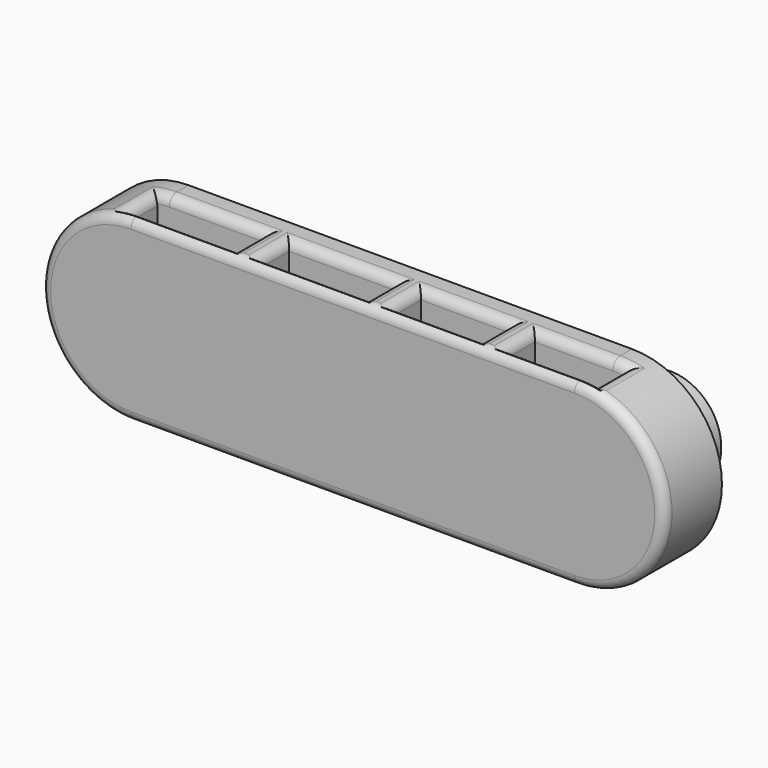
from build123d import *

# Parameters (mm, degrees)
F0_R          = 2.9
F1_DEPTH      = 2
F2_DEPTH      = 6
F3_W          = 9
F3_H          = 3
F3_W_2        = 7.5
F3_W_3        = 1
F3_W_4        = 8
F3_W_5        = 6.5
F4_DEPTH      = 15.001
F5_R          = 4.25
F5_R_2        = 2.9
F6_DEPTH      = 2
F7_T1_DEPTH   = 3
F7_T3_DEPTH   = 6.5
F7_T5_DEPTH   = 7.5
F7_T7_DEPTH   = 9
F7_T9_DEPTH   = 8
F7_T11_DEPTH  = 37
F7_T14_ANGLE  = 180
F7_T18_ANGLE  = 22.9411746719
F7_T21_ANGLE  = 180
F7_T25_ANGLE  = 22.9411746719
F7_T30_ANGLE  = 22.9411746719
F7_T35_ANGLE  = 22.9411746719
F7_T40_ANGLE  = 22.9411746719
F7_T45_ANGLE  = 22.9411746719
F7_T50_ANGLE  = 22.9411746719
F7_T55_ANGLE  = 22.9411746719
F7_T61_DEPTH  = 5.5904344641
F7_T66_ANGLE  = 22.9411746719
F7_T73_ANGLE  = 22.9411746719
F7_T77_DEPTH  = 5.5904344641
F7_T85_ANGLE  = 22.9411746719
F7_T89_DEPTH  = 5.5904344641
F7_T97_DEPTH  = 5.5904344641
F7_T102_ANGLE = 22.9411746719
F7_T109_DEPTH = 5
F7_T113_DEPTH = 8.5
F7_T120_DEPTH = 8.5
F7_T124_DEPTH = 5
F7_T132_DEPTH = 5
F7_T137_DEPTH = 9.5
F7_T144_DEPTH = 5
F7_T148_DEPTH = 9.5
F7_T155_DEPTH = 5
F7_T159_DEPTH = 9.5
F7_T166_DEPTH = 9.5
F7_T170_DEPTH = 5
F7_T178_DEPTH = 5
F7_T183_DEPTH = 11
F7_T190_DEPTH = 5
F7_T194_DEPTH = 11
F7_T201_DEPTH = 5
F7_T205_DEPTH = 11
F7_T212_DEPTH = 11
F7_T216_DEPTH = 5
F7_T224_DEPTH = 5
F7_T229_DEPTH = 10
F7_T236_DEPTH = 10
F7_T240_DEPTH = 5
F7_T247_DEPTH = 5.5904344641
F7_T252_ANGLE = 22.9411746719
F7_T259_ANGLE = 22.9411746719
F7_T263_DEPTH = 5.5904344641
F7_T271_ANGLE = 22.9411746719
F7_T275_DEPTH = 5.5904344641
F7_T283_DEPTH = 5.5904344641
F7_T288_ANGLE = 22.9411746719
F7_T295_DEPTH = 5
F7_T300_DEPTH = 8.5
F7_T307_DEPTH = 8.5
F7_T311_DEPTH = 5
F7_T318_DEPTH = 9.5
F7_T322_DEPTH = 5
F7_T330_DEPTH = 9.5
F7_T334_DEPTH = 5
F7_T341_DEPTH = 9.5
F7_T345_DEPTH = 5
F7_T352_DEPTH = 5
F7_T357_DEPTH = 9.5
F7_T364_DEPTH = 11
F7_T368_DEPTH = 5
F7_T376_DEPTH = 11
F7_T380_DEPTH = 5
F7_T387_DEPTH = 11
F7_T391_DEPTH = 5
F7_T398_DEPTH = 5
F7_T403_DEPTH = 11
F7_T410_DEPTH = 10
F7_T414_DEPTH = 5
F7_T422_DEPTH = 5
F7_T426_DEPTH = 10


# Not quite as in the source:
# - a fillet or chamfer that OpenCascade refuses, or shapes differently, is made with other operations: its cross-section is extruded or revolved along the edge and cut away or added


with BuildPart() as f1:
    # F0 (on Front) → F1 (new body)
    with BuildSketch(Plane.XZ):
        with Locations((-18.5, 0)):
            Circle(F0_R)
    extrude(amount=-F1_DEPTH)



with BuildPart() as f1b:
    # F0 (on Front) → F1, piece 2 (new body)
    with BuildSketch(Plane.XZ):
        with Locations((18.5, 0)):
            Circle(F0_R)
    extrude(amount=-F1_DEPTH)


with BuildPart() as f1_1:
    add(f1.part)

    add(f1b.part)  # F2 merges F1b
    # F0 (on Front) → F2 (join)
    with BuildSketch(Plane.XZ):
        with BuildLine():
            Line((18.5, 7.5), (-18.5, 7.5))
            ThreePointArc((-18.5, 7.5), (-26, 0), (-18.5, -7.5))
            Line((-18.5, -7.5), (18.5, -7.5))
            ThreePointArc((18.5, -7.5), (26, 0), (18.5, 7.5))
        make_face()
        with Locations((-18.5, 0)):
            Circle(F0_R, mode=Mode.SUBTRACT)
        with Locations((18.5, 0)):
            Circle(F0_R, mode=Mode.SUBTRACT)
        with Locations((-18.5, 0)):
            Circle(F0_R)
        with Locations((18.5, 0)):
            Circle(F0_R)
    extrude(amount=F2_DEPTH)

    # F3 (on face) → F4 (cut, through all)
    with BuildSketch(Plane.XY.offset(7.5)):
        with Locations((-4, -3.5)):
            Rectangle(F3_W, F3_H)
        with Locations((6.25, -3.5)):
            Rectangle(F3_W_2, F3_H)
        with Locations((-19, -3.5)):
            Rectangle(F3_W_3, F3_H)
        with Locations((-14.5, -3.5)):
            Rectangle(F3_W_4, F3_H)
        with Locations((15.25, -3.5)):
            Rectangle(F3_W_5, F3_H)
        with Locations((19, -3.5)):
            Rectangle(F3_W_3, F3_H)
    extrude(amount=-F4_DEPTH, mode=Mode.SUBTRACT)

    # F5 (on face) → F6 (join)
    with BuildSketch(Plane(origin=(0, 2, 0), x_dir=(-1, 0, 0), z_dir=(0, 1, 0))):
        with Locations((-18.5, 0)):
            Circle(F5_R)
        with Locations((18.5, 0)):
            Circle(F5_R)
        with Locations((18.5, 0)):
            Circle(F5_R_2, mode=Mode.SUBTRACT)
        with Locations((18.5, 0)):
            Circle(F5_R_2)
    extrude(amount=F6_DEPTH)

    # F7: fillet of radius 0.8 on 40 edges, made by hand

    # F7_s2 → F7_t1 (cut)
    with BuildSketch(Plane.XZ.offset(2)):
        with BuildLine():
            ThreePointArc((20.5149253731, 7.2242699106), (19.8162336817, 7.0908389885), (19.5, 6.4536811201))
            Line((19.5, 6.4536811201), (19.5, 7.4330343737))
            ThreePointArc((19.5, 7.4330343737), (20.0110722688, 7.3462004192), (20.5149253731, 7.2242699106))
        make_face()
        with BuildLine():
            ThreePointArc((20.5149253731, -7.2242699106), (19.8162336817, -7.0908389885), (19.5, -6.4536811201))
            Line((19.5, -6.4536811201), (19.5, -7.4330343737))
            ThreePointArc((19.5, -7.4330343737), (20.0110722688, -7.3462004192), (20.5149253731, -7.2242699106))
        make_face()
        with BuildLine():
            ThreePointArc((11.2, 7.5), (11.7656854249, 7.2656854249), (12, 6.7))
            Line((12, 6.7), (12, 7.5))
            Line((12, 7.5), (11.2, 7.5))
        make_face()
        with BuildLine():
            ThreePointArc((10.8, 7.5), (10.2343145751, 7.2656854249), (10, 6.7))
            Line((10, 6.7), (10, 7.5))
            Line((10, 7.5), (10.8, 7.5))
        make_face()
        with BuildLine():
            ThreePointArc((1.7, 7.5), (2.2656854249, 7.2656854249), (2.5, 6.7))
            Line((2.5, 6.7), (2.5, 7.5))
            Line((2.5, 7.5), (1.7, 7.5))
        make_face()
        with BuildLine():
            ThreePointArc((1.3, 7.5), (0.7343145751, 7.2656854249), (0.5, 6.7))
            Line((0.5, 6.7), (0.5, 7.5))
            Line((0.5, 7.5), (1.3, 7.5))
        make_face()
        with BuildLine():
            ThreePointArc((-9.3, 7.5), (-8.7343145751, 7.2656854249), (-8.5, 6.7))
            Line((-8.5, 6.7), (-8.5, 7.5))
            Line((-8.5, 7.5), (-9.3, 7.5))
        make_face()
        with BuildLine():
            ThreePointArc((-9.7, 7.5), (-10.2656854249, 7.2656854249), (-10.5, 6.7))
            Line((-10.5, 6.7), (-10.5, 7.5))
            Line((-10.5, 7.5), (-9.7, 7.5))
        make_face()
        with BuildLine():
            ThreePointArc((-20.5149253731, -7.2242699106), (-19.8162336817, -7.0908389885), (-19.5, -6.4536811201))
            Line((-19.5, -6.4536811201), (-19.5, -7.4330343737))
            ThreePointArc((-19.5, -7.4330343737), (-20.0110722688, -7.3462004192), (-20.5149253731, -7.2242699106))
        make_face()
        with BuildLine():
            ThreePointArc((-20.5149253731, 7.2242699106), (-19.8162336817, 7.0908389885), (-19.5, 6.4536811201))
            Line((-19.5, 6.4536811201), (-19.5, 7.4330343737))
            ThreePointArc((-19.5, 7.4330343737), (-20.0110722688, 7.3462004192), (-20.5149253731, 7.2242699106))
        make_face()
        with BuildLine():
            ThreePointArc((11.2, -7.5), (11.7656854249, -7.2656854249), (12, -6.7))
            Line((12, -6.7), (12, -7.5))
            Line((12, -7.5), (11.2, -7.5))
        make_face()
        with BuildLine():
            ThreePointArc((10.8, -7.5), (10.2343145751, -7.2656854249), (10, -6.7))
            Line((10, -6.7), (10, -7.5))
            Line((10, -7.5), (10.8, -7.5))
        make_face()
        with BuildLine():
            ThreePointArc((1.7, -7.5), (2.2656854249, -7.2656854249), (2.5, -6.7))
            Line((2.5, -6.7), (2.5, -7.5))
            Line((2.5, -7.5), (1.7, -7.5))
        make_face()
        with BuildLine():
            ThreePointArc((1.3, -7.5), (0.7343145751, -7.2656854249), (0.5, -6.7))
            Line((0.5, -6.7), (0.5, -7.5))
            Line((0.5, -7.5), (1.3, -7.5))
        make_face()
        with BuildLine():
            ThreePointArc((-9.3, -7.5), (-8.7343145751, -7.2656854249), (-8.5, -6.7))
            Line((-8.5, -6.7), (-8.5, -7.5))
            Line((-8.5, -7.5), (-9.3, -7.5))
        make_face()
        with BuildLine():
            ThreePointArc((-9.7, -7.5), (-10.2656854249, -7.2656854249), (-10.5, -6.7))
            Line((-10.5, -6.7), (-10.5, -7.5))
            Line((-10.5, -7.5), (-9.7, -7.5))
        make_face()
    extrude(amount=F7_T1_DEPTH, mode=Mode.SUBTRACT)

    # F7_s4 → F7_t3 (cut)
    with BuildSketch(Plane.YZ.offset(12)):
        with BuildLine():
            ThreePointArc((-5.8, 7.5), (-5.2343145751, 7.2656854249), (-5, 6.7))
            Line((-5, 6.7), (-5, 7.5))
            Line((-5, 7.5), (-5.8, 7.5))
        make_face()
        with BuildLine():
            ThreePointArc((-1.2, 7.5), (-1.7656854249, 7.2656854249), (-2, 6.7))
            Line((-2, 6.7), (-2, 7.5))
            Line((-2, 7.5), (-1.2, 7.5))
        make_face()
        with BuildLine():
            ThreePointArc((-5.8, -7.5), (-5.2343145751, -7.2656854249), (-5, -6.7))
            Line((-5, -6.7), (-5, -7.5))
            Line((-5, -7.5), (-5.8, -7.5))
        make_face()
        with BuildLine():
            ThreePointArc((-1.2, -7.5), (-1.7656854249, -7.2656854249), (-2, -6.7))
            Line((-2, -6.7), (-2, -7.5))
            Line((-2, -7.5), (-1.2, -7.5))
        make_face()
    extrude(amount=F7_T3_DEPTH, mode=Mode.SUBTRACT)

    # F7_s6 → F7_t5 (cut)
    with BuildSketch(Plane.YZ.offset(2.5)):
        with BuildLine():
            ThreePointArc((-5.8, 7.5), (-5.2343145751, 7.2656854249), (-5, 6.7))
            Line((-5, 6.7), (-5, 7.5))
            Line((-5, 7.5), (-5.8, 7.5))
        make_face()
        with BuildLine():
            ThreePointArc((-1.2, 7.5), (-1.7656854249, 7.2656854249), (-2, 6.7))
            Line((-2, 6.7), (-2, 7.5))
            Line((-2, 7.5), (-1.2, 7.5))
        make_face()
        with BuildLine():
            ThreePointArc((-1.2, -7.5), (-1.7656854249, -7.2656854249), (-2, -6.7))
            Line((-2, -6.7), (-2, -7.5))
            Line((-2, -7.5), (-1.2, -7.5))
        make_face()
        with BuildLine():
            ThreePointArc((-5.8, -7.5), (-5.2343145751, -7.2656854249), (-5, -6.7))
            Line((-5, -6.7), (-5, -7.5))
            Line((-5, -7.5), (-5.8, -7.5))
        make_face()
    extrude(amount=F7_T5_DEPTH, mode=Mode.SUBTRACT)

    # F7_s8 → F7_t7 (cut)
    with BuildSketch(Plane.YZ.offset(-8.5)):
        with BuildLine():
            ThreePointArc((-1.2, 7.5), (-1.7656854249, 7.2656854249), (-2, 6.7))
            Line((-2, 6.7), (-2, 7.5))
            Line((-2, 7.5), (-1.2, 7.5))
        make_face()
        with BuildLine():
            ThreePointArc((-5.8, 7.5), (-5.2343145751, 7.2656854249), (-5, 6.7))
            Line((-5, 6.7), (-5, 7.5))
            Line((-5, 7.5), (-5.8, 7.5))
        make_face()
        with BuildLine():
            ThreePointArc((-1.2, -7.5), (-1.7656854249, -7.2656854249), (-2, -6.7))
            Line((-2, -6.7), (-2, -7.5))
            Line((-2, -7.5), (-1.2, -7.5))
        make_face()
        with BuildLine():
            ThreePointArc((-5.8, -7.5), (-5.2343145751, -7.2656854249), (-5, -6.7))
            Line((-5, -6.7), (-5, -7.5))
            Line((-5, -7.5), (-5.8, -7.5))
        make_face()
    extrude(amount=F7_T7_DEPTH, mode=Mode.SUBTRACT)

    # F7_s10 → F7_t9 (cut)
    with BuildSketch(Plane.YZ.offset(-18.5)):
        with BuildLine():
            ThreePointArc((-5.8, 7.5), (-5.2343145751, 7.2656854249), (-5, 6.7))
            Line((-5, 6.7), (-5, 7.5))
            Line((-5, 7.5), (-5.8, 7.5))
        make_face()
        with BuildLine():
            ThreePointArc((-1.2, 7.5), (-1.7656854249, 7.2656854249), (-2, 6.7))
            Line((-2, 6.7), (-2, 7.5))
            Line((-2, 7.5), (-1.2, 7.5))
        make_face()
        with BuildLine():
            ThreePointArc((-1.2, -7.5), (-1.7656854249, -7.2656854249), (-2, -6.7))
            Line((-2, -6.7), (-2, -7.5))
            Line((-2, -7.5), (-1.2, -7.5))
        make_face()
        with BuildLine():
            ThreePointArc((-5.8, -7.5), (-5.2343145751, -7.2656854249), (-5, -6.7))
            Line((-5, -6.7), (-5, -7.5))
            Line((-5, -7.5), (-5.8, -7.5))
        make_face()
    extrude(amount=F7_T9_DEPTH, mode=Mode.SUBTRACT)

    # F7_s12 → F7_t11 (cut)
    with BuildSketch(Plane.YZ.offset(-18.5)):
        with BuildLine():
            ThreePointArc((-5.2, 7.5), (-5.7656854249, 7.2656854249), (-6, 6.7))
            Line((-6, 6.7), (-6, 7.5))
            Line((-6, 7.5), (-5.2, 7.5))
        make_face()
        with BuildLine():
            ThreePointArc((-5.2, -7.5), (-5.7656854249, -7.2656854249), (-6, -6.7))
            Line((-6, -6.7), (-6, -7.5))
            Line((-6, -7.5), (-5.2, -7.5))
        make_face()
    extrude(amount=F7_T11_DEPTH, mode=Mode.SUBTRACT)

    # F7_s13 → F7_t14 (revolve, cut)
    with BuildSketch(Plane.YZ.offset(-18.5)):
        with BuildLine():
            ThreePointArc((-5.2, 7.5), (-5.7656854249, 7.2656854249), (-6, 6.7))
            Line((-6, 6.7), (-6, 7.5))
            Line((-6, 7.5), (-5.2, 7.5))
        make_face()
    revolve(axis=Axis((-18.5, -6, 0), (0, -1, 0)), revolution_arc=F7_T14_ANGLE, mode=Mode.SUBTRACT)


with BuildPart() as f7_tool16:
    # F7_s17 → F7_t18 (revolve)
    with BuildSketch(Plane.YZ.offset(18.5)):
        with BuildLine():
            ThreePointArc((-1.2, 7.5), (-1.7656854249, 7.2656854249), (-2, 6.7))
            Line((-2, 6.7), (-2, 7.5))
            Line((-2, 7.5), (-1.2, 7.5))
        make_face()
    revolve(axis=Axis((18.5, -2, 0), (0, 1, 0)), revolution_arc=F7_T18_ANGLE)

    split(bisect_by=Plane.YZ.offset(19.5), keep=Keep.BOTTOM)


with BuildPart() as f1_2:
    add(f1_1.part)

    # F7_t15: cut F7_tool16
    add(f7_tool16.part, mode=Mode.SUBTRACT)

    # F7_s20 → F7_t21 (revolve, cut)
    with BuildSketch(Plane.YZ.offset(18.5)):
        with BuildLine():
            ThreePointArc((-5.2, -7.5), (-5.7656854249, -7.2656854249), (-6, -6.7))
            Line((-6, -6.7), (-6, -7.5))
            Line((-6, -7.5), (-5.2, -7.5))
        make_face()
    revolve(axis=Axis((18.5, -6, 0), (0, -1, 0)), revolution_arc=F7_T21_ANGLE, mode=Mode.SUBTRACT)


with BuildPart() as f7_tool23:
    # F7_s24 → F7_t25 (revolve)
    with BuildSketch(Plane(origin=(15.6892394171, 0, 6.640684884), x_dir=(0, 1, 0), z_dir=(0.9209055302, 0, 0.3897858444))):
        with BuildLine():
            ThreePointArc((-1.2, -14.7110381211), (-1.7656854249, -14.476723546), (-2, -13.9110381211))
            Line((-2, -13.9110381211), (-2, -14.7110381211))
            Line((-2, -14.7110381211), (-1.2, -14.7110381211))
        make_face()
    revolve(axis=Axis((18.5, -2, 0), (0, 1, 0)), revolution_arc=F7_T25_ANGLE)

    split(bisect_by=Plane.YZ.offset(19.5), keep=Keep.BOTTOM)


with BuildPart() as f1_3:
    add(f1_2.part)

    # F7_t22: cut F7_tool23
    add(f7_tool23.part, mode=Mode.SUBTRACT)


with BuildPart() as f7_tool28:
    # F7_s29 → F7_t30 (revolve)
    with BuildSketch(Plane.YZ.offset(-18.5)):
        with BuildLine():
            ThreePointArc((-1.2, -7.5), (-1.7656854249, -7.2656854249), (-2, -6.7))
            Line((-2, -6.7), (-2, -7.5))
            Line((-2, -7.5), (-1.2, -7.5))
        make_face()
    revolve(axis=Axis((-18.5, -2, 0), (0, 1, 0)), revolution_arc=F7_T30_ANGLE)

    split(bisect_by=Plane.YZ.offset(-19.5), keep=Keep.TOP)


with BuildPart() as f1_4:
    add(f1_3.part)

    # F7_t27: cut F7_tool28
    add(f7_tool28.part, mode=Mode.SUBTRACT)


with BuildPart() as f7_tool33:
    # F7_s34 → F7_t35 (revolve)
    with BuildSketch(Plane(origin=(-15.6892394171, 0, -6.640684884), x_dir=(0, 1, 0), z_dir=(-0.9209055302, 0, -0.3897858444))):
        with BuildLine():
            ThreePointArc((-1.2, -14.7110381211), (-1.7656854249, -14.476723546), (-2, -13.9110381211))
            Line((-2, -13.9110381211), (-2, -14.7110381211))
            Line((-2, -14.7110381211), (-1.2, -14.7110381211))
        make_face()
    revolve(axis=Axis((-18.5, -2, 0), (0, 1, 0)), revolution_arc=F7_T35_ANGLE)

    split(bisect_by=Plane.YZ.offset(-19.5), keep=Keep.TOP)


with BuildPart() as f1_5:
    add(f1_4.part)

    # F7_t32: cut F7_tool33
    add(f7_tool33.part, mode=Mode.SUBTRACT)


with BuildPart() as f7_tool38:
    # F7_s39 → F7_t40 (revolve)
    with BuildSketch(Plane.YZ.offset(-18.5)):
        with BuildLine():
            ThreePointArc((-5.8, -7.5), (-5.2343145751, -7.2656854249), (-5, -6.7))
            Line((-5, -6.7), (-5, -7.5))
            Line((-5, -7.5), (-5.8, -7.5))
        make_face()
    revolve(axis=Axis((-18.5, -5, 0), (0, 1, 0)), revolution_arc=F7_T40_ANGLE)

    split(bisect_by=Plane.YZ.offset(-19.5), keep=Keep.TOP)


with BuildPart() as f1_6:
    add(f1_5.part)

    # F7_t37: cut F7_tool38
    add(f7_tool38.part, mode=Mode.SUBTRACT)


with BuildPart() as f7_tool43:
    # F7_s44 → F7_t45 (revolve)
    with BuildSketch(Plane(origin=(15.6892394171, 0, 6.640684884), x_dir=(0, 1, 0), z_dir=(0.9209055302, 0, 0.3897858444))):
        with BuildLine():
            ThreePointArc((-5.8, -14.7110381211), (-5.2343145751, -14.476723546), (-5, -13.9110381211))
            Line((-5, -13.9110381211), (-5, -14.7110381211))
            Line((-5, -14.7110381211), (-5.8, -14.7110381211))
        make_face()
    revolve(axis=Axis((18.5, -5, 0), (0, 1, 0)), revolution_arc=F7_T45_ANGLE)

    split(bisect_by=Plane.YZ.offset(19.5), keep=Keep.BOTTOM)


with BuildPart() as f1_7:
    add(f1_6.part)

    # F7_t42: cut F7_tool43
    add(f7_tool43.part, mode=Mode.SUBTRACT)


with BuildPart() as f7_tool48:
    # F7_s49 → F7_t50 (revolve)
    with BuildSketch(Plane(origin=(-15.6892394171, 0, -6.640684884), x_dir=(0, 1, 0), z_dir=(-0.9209055302, 0, -0.3897858444))):
        with BuildLine():
            ThreePointArc((-5.8, -14.7110381211), (-5.2343145751, -14.476723546), (-5, -13.9110381211))
            Line((-5, -13.9110381211), (-5, -14.7110381211))
            Line((-5, -14.7110381211), (-5.8, -14.7110381211))
        make_face()
    revolve(axis=Axis((-18.5, -5, 0), (0, 1, 0)), revolution_arc=F7_T50_ANGLE)

    split(bisect_by=Plane.YZ.offset(-19.5), keep=Keep.TOP)


with BuildPart() as f1_8:
    add(f1_7.part)

    # F7_t47: cut F7_tool48
    add(f7_tool48.part, mode=Mode.SUBTRACT)


with BuildPart() as f7_tool53:
    # F7_s54 → F7_t55 (revolve)
    with BuildSketch(Plane.YZ.offset(18.5)):
        with BuildLine():
            ThreePointArc((-5.8, 7.5), (-5.2343145751, 7.2656854249), (-5, 6.7))
            Line((-5, 6.7), (-5, 7.5))
            Line((-5, 7.5), (-5.8, 7.5))
        make_face()
    revolve(axis=Axis((18.5, -5, 0), (0, 1, 0)), revolution_arc=F7_T55_ANGLE)

    split(bisect_by=Plane.YZ.offset(19.5), keep=Keep.BOTTOM)


with BuildPart() as f1_9:
    add(f1_8.part)

    # F7_t52: cut F7_tool53
    add(f7_tool53.part, mode=Mode.SUBTRACT)


with BuildPart() as f7_tool59:
    # F7_s60 → F7_t61 (new body)
    with BuildSketch(Plane.XZ.offset(7.5904344641)):
        with BuildLine():
            ThreePointArc((20.5149253731, 7.2242699106), (19.8162336817, 7.0908389885), (19.5, 6.4536811201))
            Line((19.5, 6.4536811201), (19.5, 7.4330343737))
            ThreePointArc((19.5, 7.4330343737), (20.0110722688, 7.3462004192), (20.5149253731, 7.2242699106))
        make_face()
    extrude(amount=-F7_T61_DEPTH)

    split(bisect_by=Plane.XZ.offset(6), keep=Keep.BOTTOM)

    split(bisect_by=Plane.XZ.offset(5), keep=Keep.TOP)


with BuildPart() as f7_tool64:
    # F7_s65 → F7_t66 (revolve)
    with BuildSketch(Plane.YZ.offset(18.5)):
        with BuildLine():
            ThreePointArc((-5.8, 7.5), (-5.2343145751, 7.2656854249), (-5, 6.7))
            Line((-5, 6.7), (-5, 7.5))
            Line((-5, 7.5), (-5.8, 7.5))
        make_face()
    revolve(axis=Axis((18.5, -5, 0), (0, 1, 0)), revolution_arc=F7_T66_ANGLE)

    split(bisect_by=Plane.YZ.offset(19.5), keep=Keep.TOP)


with BuildPart() as f7_tool59_1:
    add(f7_tool59.part)

    # F7_t68: intersect F7_tool64
    add(f7_tool64.part, mode=Mode.INTERSECT)


with BuildPart() as f1_10:
    add(f1_9.part)

    # F7_t57: cut F7_tool59
    add(f7_tool59_1.part, mode=Mode.SUBTRACT)


with BuildPart() as f7_tool71:
    # F7_s72 → F7_t73 (revolve)
    with BuildSketch(Plane.YZ.offset(18.5)):
        with BuildLine():
            ThreePointArc((-1.2, 7.5), (-1.7656854249, 7.2656854249), (-2, 6.7))
            Line((-2, 6.7), (-2, 7.5))
            Line((-2, 7.5), (-1.2, 7.5))
        make_face()
    revolve(axis=Axis((18.5, -2, 0), (0, 1, 0)), revolution_arc=F7_T73_ANGLE)

    split(bisect_by=Plane.YZ.offset(19.5), keep=Keep.TOP)


with BuildPart() as f7_tool75:
    # F7_s76 → F7_t77 (new body)
    with BuildSketch(Plane.XZ.offset(5)):
        with BuildLine():
            ThreePointArc((20.5149253731, 7.2242699106), (19.8162336817, 7.0908389885), (19.5, 6.4536811201))
            Line((19.5, 6.4536811201), (19.5, 7.4330343737))
            ThreePointArc((19.5, 7.4330343737), (20.0110722688, 7.3462004192), (20.5149253731, 7.2242699106))
        make_face()
    extrude(amount=-F7_T77_DEPTH)

    split(bisect_by=Plane.XZ, keep=Keep.TOP)

    split(bisect_by=Plane.XZ.offset(2), keep=Keep.BOTTOM)


with BuildPart() as f7_tool71_1:
    add(f7_tool71.part)

    # F7_t80: intersect F7_tool75
    add(f7_tool75.part, mode=Mode.INTERSECT)


with BuildPart() as f1_11:
    add(f1_10.part)

    # F7_t69: cut F7_tool71
    add(f7_tool71_1.part, mode=Mode.SUBTRACT)


with BuildPart() as f7_tool83:
    # F7_s84 → F7_t85 (revolve)
    with BuildSketch(Plane(origin=(15.6892394171, 0, 6.640684884), x_dir=(0, 1, 0), z_dir=(0.9209055302, 0, 0.3897858444))):
        with BuildLine():
            ThreePointArc((-5.8, -14.7110381211), (-5.2343145751, -14.476723546), (-5, -13.9110381211))
            Line((-5, -13.9110381211), (-5, -14.7110381211))
            Line((-5, -14.7110381211), (-5.8, -14.7110381211))
        make_face()
    revolve(axis=Axis((18.5, -5, 0), (0, 1, 0)), revolution_arc=F7_T85_ANGLE)

    split(bisect_by=Plane.YZ.offset(19.5), keep=Keep.TOP)


with BuildPart() as f7_tool87:
    # F7_s88 → F7_t89 (new body)
    with BuildSketch(Plane.XZ.offset(7.5904344641)):
        with BuildLine():
            ThreePointArc((20.5149253731, -7.2242699106), (19.8162336817, -7.0908389885), (19.5, -6.4536811201))
            Line((19.5, -6.4536811201), (19.5, -7.4330343737))
            ThreePointArc((19.5, -7.4330343737), (20.0110722688, -7.3462004192), (20.5149253731, -7.2242699106))
        make_face()
    extrude(amount=-F7_T89_DEPTH)

    split(bisect_by=Plane.XZ.offset(6), keep=Keep.BOTTOM)

    split(bisect_by=Plane.XZ.offset(5), keep=Keep.TOP)


with BuildPart() as f7_tool83_1:
    add(f7_tool83.part)

    # F7_t92: intersect F7_tool87
    add(f7_tool87.part, mode=Mode.INTERSECT)


with BuildPart() as f1_12:
    add(f1_11.part)

    # F7_t81: cut F7_tool83
    add(f7_tool83_1.part, mode=Mode.SUBTRACT)


with BuildPart() as f7_tool95:
    # F7_s96 → F7_t97 (new body)
    with BuildSketch(Plane.XZ.offset(5)):
        with BuildLine():
            ThreePointArc((20.5149253731, -7.2242699106), (19.8162336817, -7.0908389885), (19.5, -6.4536811201))
            Line((19.5, -6.4536811201), (19.5, -7.4330343737))
            ThreePointArc((19.5, -7.4330343737), (20.0110722688, -7.3462004192), (20.5149253731, -7.2242699106))
        make_face()
    extrude(amount=-F7_T97_DEPTH)

    split(bisect_by=Plane.XZ, keep=Keep.TOP)

    split(bisect_by=Plane.XZ.offset(2), keep=Keep.BOTTOM)


with BuildPart() as f7_tool100:
    # F7_s101 → F7_t102 (revolve)
    with BuildSketch(Plane(origin=(15.6892394171, 0, 6.640684884), x_dir=(0, 1, 0), z_dir=(0.9209055302, 0, 0.3897858444))):
        with BuildLine():
            ThreePointArc((-1.2, -14.7110381211), (-1.7656854249, -14.476723546), (-2, -13.9110381211))
            Line((-2, -13.9110381211), (-2, -14.7110381211))
            Line((-2, -14.7110381211), (-1.2, -14.7110381211))
        make_face()
    revolve(axis=Axis((18.5, -2, 0), (0, 1, 0)), revolution_arc=F7_T102_ANGLE)

    split(bisect_by=Plane.YZ.offset(19.5), keep=Keep.TOP)


with BuildPart() as f7_tool95_1:
    add(f7_tool95.part)

    # F7_t104: intersect F7_tool100
    add(f7_tool100.part, mode=Mode.INTERSECT)


with BuildPart() as f1_13:
    add(f1_12.part)

    # F7_t93: cut F7_tool95
    add(f7_tool95_1.part, mode=Mode.SUBTRACT)


with BuildPart() as f7_tool107:
    # F7_s108 → F7_t109 (new body)
    with BuildSketch(Plane.XZ):
        with BuildLine():
            ThreePointArc((11.2, 7.5), (11.7656854249, 7.2656854249), (12, 6.7))
            Line((12, 6.7), (12, 7.5))
            Line((12, 7.5), (11.2, 7.5))
        make_face()
    extrude(amount=F7_T109_DEPTH)

    split(bisect_by=Plane.XZ.offset(2), keep=Keep.BOTTOM)


with BuildPart() as f7_tool111:
    # F7_s112 → F7_t113 (new body)
    with BuildSketch(Plane.YZ.offset(18.5)):
        with BuildLine():
            ThreePointArc((-1.2, 7.5), (-1.7656854249, 7.2656854249), (-2, 6.7))
            Line((-2, 6.7), (-2, 7.5))
            Line((-2, 7.5), (-1.2, 7.5))
        make_face()
    extrude(amount=-F7_T113_DEPTH)

    split(bisect_by=Plane.YZ.offset(12), keep=Keep.BOTTOM)


with BuildPart() as f7_tool107_1:
    add(f7_tool107.part)

    # F7_t115: intersect F7_tool111
    add(f7_tool111.part, mode=Mode.INTERSECT)


with BuildPart() as f1_14:
    add(f1_13.part)

    # F7_t105: cut F7_tool107
    add(f7_tool107_1.part, mode=Mode.SUBTRACT)


with BuildPart() as f7_tool118:
    # F7_s119 → F7_t120 (new body)
    with BuildSketch(Plane.YZ.offset(10)):
        with BuildLine():
            ThreePointArc((-5.8, 7.5), (-5.2343145751, 7.2656854249), (-5, 6.7))
            Line((-5, 6.7), (-5, 7.5))
            Line((-5, 7.5), (-5.8, 7.5))
        make_face()
    extrude(amount=F7_T120_DEPTH)

    split(bisect_by=Plane.YZ.offset(12), keep=Keep.BOTTOM)


with BuildPart() as f7_tool122:
    # F7_s123 → F7_t124 (new body)
    with BuildSketch(Plane.XZ.offset(2)):
        with BuildLine():
            ThreePointArc((11.2, 7.5), (11.7656854249, 7.2656854249), (12, 6.7))
            Line((12, 6.7), (12, 7.5))
            Line((12, 7.5), (11.2, 7.5))
        make_face()
    extrude(amount=F7_T124_DEPTH)

    split(bisect_by=Plane.XZ.offset(6), keep=Keep.BOTTOM)

    split(bisect_by=Plane.XZ.offset(5), keep=Keep.TOP)


with BuildPart() as f7_tool118_1:
    add(f7_tool118.part)

    # F7_t127: intersect F7_tool122
    add(f7_tool122.part, mode=Mode.INTERSECT)


with BuildPart() as f1_15:
    add(f1_14.part)

    # F7_t116: cut F7_tool118
    add(f7_tool118_1.part, mode=Mode.SUBTRACT)


with BuildPart() as f7_tool130:
    # F7_s131 → F7_t132 (new body)
    with BuildSketch(Plane.XZ.offset(7)):
        with BuildLine():
            ThreePointArc((10.8, 7.5), (10.2343145751, 7.2656854249), (10, 6.7))
            Line((10, 6.7), (10, 7.5))
            Line((10, 7.5), (10.8, 7.5))
        make_face()
    extrude(amount=-F7_T132_DEPTH)

    split(bisect_by=Plane.XZ.offset(6), keep=Keep.BOTTOM)

    split(bisect_by=Plane.XZ.offset(5), keep=Keep.TOP)


with BuildPart() as f7_tool135:
    # F7_s136 → F7_t137 (new body)
    with BuildSketch(Plane.YZ.offset(2.5)):
        with BuildLine():
            ThreePointArc((-5.8, 7.5), (-5.2343145751, 7.2656854249), (-5, 6.7))
            Line((-5, 6.7), (-5, 7.5))
            Line((-5, 7.5), (-5.8, 7.5))
        make_face()
    extrude(amount=F7_T137_DEPTH)

    split(bisect_by=Plane.YZ.offset(10), keep=Keep.TOP)


with BuildPart() as f7_tool130_1:
    add(f7_tool130.part)

    # F7_t139: intersect F7_tool135
    add(f7_tool135.part, mode=Mode.INTERSECT)


with BuildPart() as f1_16:
    add(f1_15.part)

    # F7_t128: cut F7_tool130
    add(f7_tool130_1.part, mode=Mode.SUBTRACT)


with BuildPart() as f7_tool142:
    # F7_s143 → F7_t144 (new body)
    with BuildSketch(Plane.XZ.offset(5)):
        with BuildLine():
            ThreePointArc((10.8, 7.5), (10.2343145751, 7.2656854249), (10, 6.7))
            Line((10, 6.7), (10, 7.5))
            Line((10, 7.5), (10.8, 7.5))
        make_face()
    extrude(amount=-F7_T144_DEPTH)

    split(bisect_by=Plane.XZ.offset(2), keep=Keep.BOTTOM)


with BuildPart() as f7_tool146:
    # F7_s147 → F7_t148 (new body)
    with BuildSketch(Plane.YZ.offset(12)):
        with BuildLine():
            ThreePointArc((-1.2, 7.5), (-1.7656854249, 7.2656854249), (-2, 6.7))
            Line((-2, 6.7), (-2, 7.5))
            Line((-2, 7.5), (-1.2, 7.5))
        make_face()
    extrude(amount=-F7_T148_DEPTH)

    split(bisect_by=Plane.YZ.offset(10), keep=Keep.TOP)


with BuildPart() as f7_tool142_1:
    add(f7_tool142.part)

    # F7_t150: intersect F7_tool146
    add(f7_tool146.part, mode=Mode.INTERSECT)


with BuildPart() as f1_17:
    add(f1_16.part)

    # F7_t140: cut F7_tool142
    add(f7_tool142_1.part, mode=Mode.SUBTRACT)


with BuildPart() as f7_tool153:
    # F7_s154 → F7_t155 (new body)
    with BuildSketch(Plane.XZ):
        with BuildLine():
            ThreePointArc((1.7, 7.5), (2.2656854249, 7.2656854249), (2.5, 6.7))
            Line((2.5, 6.7), (2.5, 7.5))
            Line((2.5, 7.5), (1.7, 7.5))
        make_face()
    extrude(amount=F7_T155_DEPTH)

    split(bisect_by=Plane.XZ.offset(2), keep=Keep.BOTTOM)


with BuildPart() as f7_tool157:
    # F7_s158 → F7_t159 (new body)
    with BuildSketch(Plane.YZ.offset(10)):
        with BuildLine():
            ThreePointArc((-1.2, 7.5), (-1.7656854249, 7.2656854249), (-2, 6.7))
            Line((-2, 6.7), (-2, 7.5))
            Line((-2, 7.5), (-1.2, 7.5))
        make_face()
    extrude(amount=-F7_T159_DEPTH)

    split(bisect_by=Plane.YZ.offset(2.5), keep=Keep.BOTTOM)


with BuildPart() as f7_tool153_1:
    add(f7_tool153.part)

    # F7_t161: intersect F7_tool157
    add(f7_tool157.part, mode=Mode.INTERSECT)


with BuildPart() as f1_18:
    add(f1_17.part)

    # F7_t151: cut F7_tool153
    add(f7_tool153_1.part, mode=Mode.SUBTRACT)


with BuildPart() as f7_tool164:
    # F7_s165 → F7_t166 (new body)
    with BuildSketch(Plane.YZ.offset(0.5)):
        with BuildLine():
            ThreePointArc((-5.8, 7.5), (-5.2343145751, 7.2656854249), (-5, 6.7))
            Line((-5, 6.7), (-5, 7.5))
            Line((-5, 7.5), (-5.8, 7.5))
        make_face()
    extrude(amount=F7_T166_DEPTH)

    split(bisect_by=Plane.YZ.offset(2.5), keep=Keep.BOTTOM)


with BuildPart() as f7_tool168:
    # F7_s169 → F7_t170 (new body)
    with BuildSketch(Plane.XZ.offset(2)):
        with BuildLine():
            ThreePointArc((1.7, 7.5), (2.2656854249, 7.2656854249), (2.5, 6.7))
            Line((2.5, 6.7), (2.5, 7.5))
            Line((2.5, 7.5), (1.7, 7.5))
        make_face()
    extrude(amount=F7_T170_DEPTH)

    split(bisect_by=Plane.XZ.offset(6), keep=Keep.BOTTOM)

    split(bisect_by=Plane.XZ.offset(5), keep=Keep.TOP)


with BuildPart() as f7_tool164_1:
    add(f7_tool164.part)

    # F7_t173: intersect F7_tool168
    add(f7_tool168.part, mode=Mode.INTERSECT)


with BuildPart() as f1_19:
    add(f1_18.part)

    # F7_t162: cut F7_tool164
    add(f7_tool164_1.part, mode=Mode.SUBTRACT)


with BuildPart() as f7_tool176:
    # F7_s177 → F7_t178 (new body)
    with BuildSketch(Plane.XZ.offset(7)):
        with BuildLine():
            ThreePointArc((1.3, 7.5), (0.7343145751, 7.2656854249), (0.5, 6.7))
            Line((0.5, 6.7), (0.5, 7.5))
            Line((0.5, 7.5), (1.3, 7.5))
        make_face()
    extrude(amount=-F7_T178_DEPTH)

    split(bisect_by=Plane.XZ.offset(6), keep=Keep.BOTTOM)

    split(bisect_by=Plane.XZ.offset(5), keep=Keep.TOP)


with BuildPart() as f7_tool181:
    # F7_s182 → F7_t183 (new body)
    with BuildSketch(Plane.YZ.offset(-8.5)):
        with BuildLine():
            ThreePointArc((-5.8, 7.5), (-5.2343145751, 7.2656854249), (-5, 6.7))
            Line((-5, 6.7), (-5, 7.5))
            Line((-5, 7.5), (-5.8, 7.5))
        make_face()
    extrude(amount=F7_T183_DEPTH)

    split(bisect_by=Plane.YZ.offset(0.5), keep=Keep.TOP)


with BuildPart() as f7_tool176_1:
    add(f7_tool176.part)

    # F7_t185: intersect F7_tool181
    add(f7_tool181.part, mode=Mode.INTERSECT)


with BuildPart() as f1_20:
    add(f1_19.part)

    # F7_t174: cut F7_tool176
    add(f7_tool176_1.part, mode=Mode.SUBTRACT)


with BuildPart() as f7_tool188:
    # F7_s189 → F7_t190 (new body)
    with BuildSketch(Plane.XZ.offset(5)):
        with BuildLine():
            ThreePointArc((1.3, 7.5), (0.7343145751, 7.2656854249), (0.5, 6.7))
            Line((0.5, 6.7), (0.5, 7.5))
            Line((0.5, 7.5), (1.3, 7.5))
        make_face()
    extrude(amount=-F7_T190_DEPTH)

    split(bisect_by=Plane.XZ.offset(2), keep=Keep.BOTTOM)


with BuildPart() as f7_tool192:
    # F7_s193 → F7_t194 (new body)
    with BuildSketch(Plane.YZ.offset(2.5)):
        with BuildLine():
            ThreePointArc((-1.2, 7.5), (-1.7656854249, 7.2656854249), (-2, 6.7))
            Line((-2, 6.7), (-2, 7.5))
            Line((-2, 7.5), (-1.2, 7.5))
        make_face()
    extrude(amount=-F7_T194_DEPTH)

    split(bisect_by=Plane.YZ.offset(0.5), keep=Keep.TOP)


with BuildPart() as f7_tool188_1:
    add(f7_tool188.part)

    # F7_t196: intersect F7_tool192
    add(f7_tool192.part, mode=Mode.INTERSECT)


with BuildPart() as f1_21:
    add(f1_20.part)

    # F7_t186: cut F7_tool188
    add(f7_tool188_1.part, mode=Mode.SUBTRACT)


with BuildPart() as f7_tool199:
    # F7_s200 → F7_t201 (new body)
    with BuildSketch(Plane.XZ):
        with BuildLine():
            ThreePointArc((-9.3, 7.5), (-8.7343145751, 7.2656854249), (-8.5, 6.7))
            Line((-8.5, 6.7), (-8.5, 7.5))
            Line((-8.5, 7.5), (-9.3, 7.5))
        make_face()
    extrude(amount=F7_T201_DEPTH)

    split(bisect_by=Plane.XZ.offset(2), keep=Keep.BOTTOM)


with BuildPart() as f7_tool203:
    # F7_s204 → F7_t205 (new body)
    with BuildSketch(Plane.YZ.offset(0.5)):
        with BuildLine():
            ThreePointArc((-1.2, 7.5), (-1.7656854249, 7.2656854249), (-2, 6.7))
            Line((-2, 6.7), (-2, 7.5))
            Line((-2, 7.5), (-1.2, 7.5))
        make_face()
    extrude(amount=-F7_T205_DEPTH)

    split(bisect_by=Plane.YZ.offset(-8.5), keep=Keep.BOTTOM)


with BuildPart() as f7_tool199_1:
    add(f7_tool199.part)

    # F7_t207: intersect F7_tool203
    add(f7_tool203.part, mode=Mode.INTERSECT)


with BuildPart() as f1_22:
    add(f1_21.part)

    # F7_t197: cut F7_tool199
    add(f7_tool199_1.part, mode=Mode.SUBTRACT)


with BuildPart() as f7_tool210:
    # F7_s211 → F7_t212 (new body)
    with BuildSketch(Plane.YZ.offset(-10.5)):
        with BuildLine():
            ThreePointArc((-5.8, 7.5), (-5.2343145751, 7.2656854249), (-5, 6.7))
            Line((-5, 6.7), (-5, 7.5))
            Line((-5, 7.5), (-5.8, 7.5))
        make_face()
    extrude(amount=F7_T212_DEPTH)

    split(bisect_by=Plane.YZ.offset(-8.5), keep=Keep.BOTTOM)


with BuildPart() as f7_tool214:
    # F7_s215 → F7_t216 (new body)
    with BuildSketch(Plane.XZ.offset(2)):
        with BuildLine():
            ThreePointArc((-9.3, 7.5), (-8.7343145751, 7.2656854249), (-8.5, 6.7))
            Line((-8.5, 6.7), (-8.5, 7.5))
            Line((-8.5, 7.5), (-9.3, 7.5))
        make_face()
    extrude(amount=F7_T216_DEPTH)

    split(bisect_by=Plane.XZ.offset(6), keep=Keep.BOTTOM)

    split(bisect_by=Plane.XZ.offset(5), keep=Keep.TOP)


with BuildPart() as f7_tool210_1:
    add(f7_tool210.part)

    # F7_t219: intersect F7_tool214
    add(f7_tool214.part, mode=Mode.INTERSECT)


with BuildPart() as f1_23:
    add(f1_22.part)

    # F7_t208: cut F7_tool210
    add(f7_tool210_1.part, mode=Mode.SUBTRACT)


with BuildPart() as f7_tool222:
    # F7_s223 → F7_t224 (new body)
    with BuildSketch(Plane.XZ.offset(7)):
        with BuildLine():
            ThreePointArc((-9.7, 7.5), (-10.2656854249, 7.2656854249), (-10.5, 6.7))
            Line((-10.5, 6.7), (-10.5, 7.5))
            Line((-10.5, 7.5), (-9.7, 7.5))
        make_face()
    extrude(amount=-F7_T224_DEPTH)

    split(bisect_by=Plane.XZ.offset(5), keep=Keep.TOP)

    split(bisect_by=Plane.XZ.offset(6), keep=Keep.BOTTOM)


with BuildPart() as f7_tool227:
    # F7_s228 → F7_t229 (new body)
    with BuildSketch(Plane.YZ.offset(-18.5)):
        with BuildLine():
            ThreePointArc((-5.8, 7.5), (-5.2343145751, 7.2656854249), (-5, 6.7))
            Line((-5, 6.7), (-5, 7.5))
            Line((-5, 7.5), (-5.8, 7.5))
        make_face()
    extrude(amount=F7_T229_DEPTH)

    split(bisect_by=Plane.YZ.offset(-10.5), keep=Keep.TOP)


with BuildPart() as f7_tool222_1:
    add(f7_tool222.part)

    # F7_t231: intersect F7_tool227
    add(f7_tool227.part, mode=Mode.INTERSECT)


with BuildPart() as f1_24:
    add(f1_23.part)

    # F7_t220: cut F7_tool222
    add(f7_tool222_1.part, mode=Mode.SUBTRACT)


with BuildPart() as f7_tool234:
    # F7_s235 → F7_t236 (new body)
    with BuildSketch(Plane.YZ.offset(-8.5)):
        with BuildLine():
            ThreePointArc((-1.2, 7.5), (-1.7656854249, 7.2656854249), (-2, 6.7))
            Line((-2, 6.7), (-2, 7.5))
            Line((-2, 7.5), (-1.2, 7.5))
        make_face()
    extrude(amount=-F7_T236_DEPTH)

    split(bisect_by=Plane.YZ.offset(-10.5), keep=Keep.TOP)


with BuildPart() as f7_tool238:
    # F7_s239 → F7_t240 (new body)
    with BuildSketch(Plane.XZ.offset(5)):
        with BuildLine():
            ThreePointArc((-9.7, 7.5), (-10.2656854249, 7.2656854249), (-10.5, 6.7))
            Line((-10.5, 6.7), (-10.5, 7.5))
            Line((-10.5, 7.5), (-9.7, 7.5))
        make_face()
    extrude(amount=-F7_T240_DEPTH)

    split(bisect_by=Plane.XZ.offset(2), keep=Keep.BOTTOM)


with BuildPart() as f7_tool234_1:
    add(f7_tool234.part)

    # F7_t242: intersect F7_tool238
    add(f7_tool238.part, mode=Mode.INTERSECT)


with BuildPart() as f1_25:
    add(f1_24.part)

    # F7_t232: cut F7_tool234
    add(f7_tool234_1.part, mode=Mode.SUBTRACT)


with BuildPart() as f7_tool245:
    # F7_s246 → F7_t247 (new body)
    with BuildSketch(Plane.XZ.offset(7.5904344641)):
        with BuildLine():
            ThreePointArc((-20.5149253731, -7.2242699106), (-19.8162336817, -7.0908389885), (-19.5, -6.4536811201))
            Line((-19.5, -6.4536811201), (-19.5, -7.4330343737))
            ThreePointArc((-19.5, -7.4330343737), (-20.0110722688, -7.3462004192), (-20.5149253731, -7.2242699106))
        make_face()
    extrude(amount=-F7_T247_DEPTH)

    split(bisect_by=Plane.XZ.offset(5), keep=Keep.TOP)

    split(bisect_by=Plane.XZ.offset(6), keep=Keep.BOTTOM)


with BuildPart() as f7_tool250:
    # F7_s251 → F7_t252 (revolve)
    with BuildSketch(Plane.YZ.offset(-18.5)):
        with BuildLine():
            ThreePointArc((-5.8, -7.5), (-5.2343145751, -7.2656854249), (-5, -6.7))
            Line((-5, -6.7), (-5, -7.5))
            Line((-5, -7.5), (-5.8, -7.5))
        make_face()
    revolve(axis=Axis((-18.5, -5, 0), (0, 1, 0)), revolution_arc=F7_T252_ANGLE)

    split(bisect_by=Plane.YZ.offset(-19.5), keep=Keep.BOTTOM)


with BuildPart() as f7_tool245_1:
    add(f7_tool245.part)

    # F7_t254: intersect F7_tool250
    add(f7_tool250.part, mode=Mode.INTERSECT)


with BuildPart() as f1_26:
    add(f1_25.part)

    # F7_t243: cut F7_tool245
    add(f7_tool245_1.part, mode=Mode.SUBTRACT)


with BuildPart() as f7_tool257:
    # F7_s258 → F7_t259 (revolve)
    with BuildSketch(Plane.YZ.offset(-18.5)):
        with BuildLine():
            ThreePointArc((-1.2, -7.5), (-1.7656854249, -7.2656854249), (-2, -6.7))
            Line((-2, -6.7), (-2, -7.5))
            Line((-2, -7.5), (-1.2, -7.5))
        make_face()
    revolve(axis=Axis((-18.5, -2, 0), (0, 1, 0)), revolution_arc=F7_T259_ANGLE)

    split(bisect_by=Plane.YZ.offset(-19.5), keep=Keep.BOTTOM)


with BuildPart() as f7_tool261:
    # F7_s262 → F7_t263 (new body)
    with BuildSketch(Plane.XZ.offset(5)):
        with BuildLine():
            ThreePointArc((-20.5149253731, -7.2242699106), (-19.8162336817, -7.0908389885), (-19.5, -6.4536811201))
            Line((-19.5, -6.4536811201), (-19.5, -7.4330343737))
            ThreePointArc((-19.5, -7.4330343737), (-20.0110722688, -7.3462004192), (-20.5149253731, -7.2242699106))
        make_face()
    extrude(amount=-F7_T263_DEPTH)

    split(bisect_by=Plane.XZ, keep=Keep.TOP)

    split(bisect_by=Plane.XZ.offset(2), keep=Keep.BOTTOM)


with BuildPart() as f7_tool257_1:
    add(f7_tool257.part)

    # F7_t266: intersect F7_tool261
    add(f7_tool261.part, mode=Mode.INTERSECT)


with BuildPart() as f1_27:
    add(f1_26.part)

    # F7_t255: cut F7_tool257
    add(f7_tool257_1.part, mode=Mode.SUBTRACT)


with BuildPart() as f7_tool269:
    # F7_s270 → F7_t271 (revolve)
    with BuildSketch(Plane(origin=(-15.6892394171, 0, -6.640684884), x_dir=(0, 1, 0), z_dir=(-0.9209055302, 0, -0.3897858444))):
        with BuildLine():
            ThreePointArc((-5.8, -14.7110381211), (-5.2343145751, -14.476723546), (-5, -13.9110381211))
            Line((-5, -13.9110381211), (-5, -14.7110381211))
            Line((-5, -14.7110381211), (-5.8, -14.7110381211))
        make_face()
    revolve(axis=Axis((-18.5, -5, 0), (0, 1, 0)), revolution_arc=F7_T271_ANGLE)

    split(bisect_by=Plane.YZ.offset(-19.5), keep=Keep.BOTTOM)


with BuildPart() as f7_tool273:
    # F7_s274 → F7_t275 (new body)
    with BuildSketch(Plane.XZ.offset(7.5904344641)):
        with BuildLine():
            ThreePointArc((-20.5149253731, 7.2242699106), (-19.8162336817, 7.0908389885), (-19.5, 6.4536811201))
            Line((-19.5, 6.4536811201), (-19.5, 7.4330343737))
            ThreePointArc((-19.5, 7.4330343737), (-20.0110722688, 7.3462004192), (-20.5149253731, 7.2242699106))
        make_face()
    extrude(amount=-F7_T275_DEPTH)

    split(bisect_by=Plane.XZ.offset(5), keep=Keep.TOP)

    split(bisect_by=Plane.XZ.offset(6), keep=Keep.BOTTOM)


with BuildPart() as f7_tool269_1:
    add(f7_tool269.part)

    # F7_t278: intersect F7_tool273
    add(f7_tool273.part, mode=Mode.INTERSECT)


with BuildPart() as f1_28:
    add(f1_27.part)

    # F7_t267: cut F7_tool269
    add(f7_tool269_1.part, mode=Mode.SUBTRACT)


with BuildPart() as f7_tool281:
    # F7_s282 → F7_t283 (new body)
    with BuildSketch(Plane.XZ.offset(5)):
        with BuildLine():
            ThreePointArc((-20.5149253731, 7.2242699106), (-19.8162336817, 7.0908389885), (-19.5, 6.4536811201))
            Line((-19.5, 6.4536811201), (-19.5, 7.4330343737))
            ThreePointArc((-19.5, 7.4330343737), (-20.0110722688, 7.3462004192), (-20.5149253731, 7.2242699106))
        make_face()
    extrude(amount=-F7_T283_DEPTH)

    split(bisect_by=Plane.XZ, keep=Keep.TOP)

    split(bisect_by=Plane.XZ.offset(2), keep=Keep.BOTTOM)


with BuildPart() as f7_tool286:
    # F7_s287 → F7_t288 (revolve)
    with BuildSketch(Plane(origin=(-15.6892394171, 0, -6.640684884), x_dir=(0, 1, 0), z_dir=(-0.9209055302, 0, -0.3897858444))):
        with BuildLine():
            ThreePointArc((-1.2, -14.7110381211), (-1.7656854249, -14.476723546), (-2, -13.9110381211))
            Line((-2, -13.9110381211), (-2, -14.7110381211))
            Line((-2, -14.7110381211), (-1.2, -14.7110381211))
        make_face()
    revolve(axis=Axis((-18.5, -2, 0), (0, 1, 0)), revolution_arc=F7_T288_ANGLE)

    split(bisect_by=Plane.YZ.offset(-19.5), keep=Keep.BOTTOM)


with BuildPart() as f7_tool281_1:
    add(f7_tool281.part)

    # F7_t290: intersect F7_tool286
    add(f7_tool286.part, mode=Mode.INTERSECT)


with BuildPart() as f1_29:
    add(f1_28.part)

    # F7_t279: cut F7_tool281
    add(f7_tool281_1.part, mode=Mode.SUBTRACT)


with BuildPart() as f7_tool293:
    # F7_s294 → F7_t295 (new body)
    with BuildSketch(Plane.XZ.offset(2)):
        with BuildLine():
            ThreePointArc((11.2, -7.5), (11.7656854249, -7.2656854249), (12, -6.7))
            Line((12, -6.7), (12, -7.5))
            Line((12, -7.5), (11.2, -7.5))
        make_face()
    extrude(amount=F7_T295_DEPTH)

    split(bisect_by=Plane.XZ.offset(6), keep=Keep.BOTTOM)

    split(bisect_by=Plane.XZ.offset(5), keep=Keep.TOP)


with BuildPart() as f7_tool298:
    # F7_s299 → F7_t300 (new body)
    with BuildSketch(Plane.YZ.offset(10)):
        with BuildLine():
            ThreePointArc((-5.8, -7.5), (-5.2343145751, -7.2656854249), (-5, -6.7))
            Line((-5, -6.7), (-5, -7.5))
            Line((-5, -7.5), (-5.8, -7.5))
        make_face()
    extrude(amount=F7_T300_DEPTH)

    split(bisect_by=Plane.YZ.offset(12), keep=Keep.BOTTOM)


with BuildPart() as f7_tool293_1:
    add(f7_tool293.part)

    # F7_t302: intersect F7_tool298
    add(f7_tool298.part, mode=Mode.INTERSECT)


with BuildPart() as f1_30:
    add(f1_29.part)

    # F7_t291: cut F7_tool293
    add(f7_tool293_1.part, mode=Mode.SUBTRACT)


with BuildPart() as f7_tool305:
    # F7_s306 → F7_t307 (new body)
    with BuildSketch(Plane.YZ.offset(18.5)):
        with BuildLine():
            ThreePointArc((-1.2, -7.5), (-1.7656854249, -7.2656854249), (-2, -6.7))
            Line((-2, -6.7), (-2, -7.5))
            Line((-2, -7.5), (-1.2, -7.5))
        make_face()
    extrude(amount=-F7_T307_DEPTH)

    split(bisect_by=Plane.YZ.offset(12), keep=Keep.BOTTOM)


with BuildPart() as f7_tool309:
    # F7_s310 → F7_t311 (new body)
    with BuildSketch(Plane.XZ):
        with BuildLine():
            ThreePointArc((11.2, -7.5), (11.7656854249, -7.2656854249), (12, -6.7))
            Line((12, -6.7), (12, -7.5))
            Line((12, -7.5), (11.2, -7.5))
        make_face()
    extrude(amount=F7_T311_DEPTH)

    split(bisect_by=Plane.XZ.offset(2), keep=Keep.BOTTOM)


with BuildPart() as f7_tool305_1:
    add(f7_tool305.part)

    # F7_t313: intersect F7_tool309
    add(f7_tool309.part, mode=Mode.INTERSECT)


with BuildPart() as f1_31:
    add(f1_30.part)

    # F7_t303: cut F7_tool305
    add(f7_tool305_1.part, mode=Mode.SUBTRACT)


with BuildPart() as f7_tool316:
    # F7_s317 → F7_t318 (new body)
    with BuildSketch(Plane.YZ.offset(2.5)):
        with BuildLine():
            ThreePointArc((-5.8, -7.5), (-5.2343145751, -7.2656854249), (-5, -6.7))
            Line((-5, -6.7), (-5, -7.5))
            Line((-5, -7.5), (-5.8, -7.5))
        make_face()
    extrude(amount=F7_T318_DEPTH)

    split(bisect_by=Plane.YZ.offset(10), keep=Keep.TOP)


with BuildPart() as f7_tool320:
    # F7_s321 → F7_t322 (new body)
    with BuildSketch(Plane.XZ.offset(7)):
        with BuildLine():
            ThreePointArc((10.8, -7.5), (10.2343145751, -7.2656854249), (10, -6.7))
            Line((10, -6.7), (10, -7.5))
            Line((10, -7.5), (10.8, -7.5))
        make_face()
    extrude(amount=-F7_T322_DEPTH)

    split(bisect_by=Plane.XZ.offset(6), keep=Keep.BOTTOM)

    split(bisect_by=Plane.XZ.offset(5), keep=Keep.TOP)


with BuildPart() as f7_tool316_1:
    add(f7_tool316.part)

    # F7_t325: intersect F7_tool320
    add(f7_tool320.part, mode=Mode.INTERSECT)


with BuildPart() as f1_32:
    add(f1_31.part)

    # F7_t314: cut F7_tool316
    add(f7_tool316_1.part, mode=Mode.SUBTRACT)


with BuildPart() as f7_tool328:
    # F7_s329 → F7_t330 (new body)
    with BuildSketch(Plane.YZ.offset(12)):
        with BuildLine():
            ThreePointArc((-1.2, -7.5), (-1.7656854249, -7.2656854249), (-2, -6.7))
            Line((-2, -6.7), (-2, -7.5))
            Line((-2, -7.5), (-1.2, -7.5))
        make_face()
    extrude(amount=-F7_T330_DEPTH)

    split(bisect_by=Plane.YZ.offset(10), keep=Keep.TOP)


with BuildPart() as f7_tool332:
    # F7_s333 → F7_t334 (new body)
    with BuildSketch(Plane.XZ.offset(5)):
        with BuildLine():
            ThreePointArc((10.8, -7.5), (10.2343145751, -7.2656854249), (10, -6.7))
            Line((10, -6.7), (10, -7.5))
            Line((10, -7.5), (10.8, -7.5))
        make_face()
    extrude(amount=-F7_T334_DEPTH)

    split(bisect_by=Plane.XZ.offset(2), keep=Keep.BOTTOM)


with BuildPart() as f7_tool328_1:
    add(f7_tool328.part)

    # F7_t336: intersect F7_tool332
    add(f7_tool332.part, mode=Mode.INTERSECT)


with BuildPart() as f1_33:
    add(f1_32.part)

    # F7_t326: cut F7_tool328
    add(f7_tool328_1.part, mode=Mode.SUBTRACT)


with BuildPart() as f7_tool339:
    # F7_s340 → F7_t341 (new body)
    with BuildSketch(Plane.YZ.offset(10)):
        with BuildLine():
            ThreePointArc((-1.2, -7.5), (-1.7656854249, -7.2656854249), (-2, -6.7))
            Line((-2, -6.7), (-2, -7.5))
            Line((-2, -7.5), (-1.2, -7.5))
        make_face()
    extrude(amount=-F7_T341_DEPTH)

    split(bisect_by=Plane.YZ.offset(2.5), keep=Keep.BOTTOM)


with BuildPart() as f7_tool343:
    # F7_s344 → F7_t345 (new body)
    with BuildSketch(Plane.XZ):
        with BuildLine():
            ThreePointArc((1.7, -7.5), (2.2656854249, -7.2656854249), (2.5, -6.7))
            Line((2.5, -6.7), (2.5, -7.5))
            Line((2.5, -7.5), (1.7, -7.5))
        make_face()
    extrude(amount=F7_T345_DEPTH)

    split(bisect_by=Plane.XZ.offset(2), keep=Keep.BOTTOM)


with BuildPart() as f7_tool339_1:
    add(f7_tool339.part)

    # F7_t347: intersect F7_tool343
    add(f7_tool343.part, mode=Mode.INTERSECT)


with BuildPart() as f1_34:
    add(f1_33.part)

    # F7_t337: cut F7_tool339
    add(f7_tool339_1.part, mode=Mode.SUBTRACT)


with BuildPart() as f7_tool350:
    # F7_s351 → F7_t352 (new body)
    with BuildSketch(Plane.XZ.offset(2)):
        with BuildLine():
            ThreePointArc((1.7, -7.5), (2.2656854249, -7.2656854249), (2.5, -6.7))
            Line((2.5, -6.7), (2.5, -7.5))
            Line((2.5, -7.5), (1.7, -7.5))
        make_face()
    extrude(amount=F7_T352_DEPTH)

    split(bisect_by=Plane.XZ.offset(6), keep=Keep.BOTTOM)

    split(bisect_by=Plane.XZ.offset(5), keep=Keep.TOP)


with BuildPart() as f7_tool355:
    # F7_s356 → F7_t357 (new body)
    with BuildSketch(Plane.YZ.offset(0.5)):
        with BuildLine():
            ThreePointArc((-5.8, -7.5), (-5.2343145751, -7.2656854249), (-5, -6.7))
            Line((-5, -6.7), (-5, -7.5))
            Line((-5, -7.5), (-5.8, -7.5))
        make_face()
    extrude(amount=F7_T357_DEPTH)

    split(bisect_by=Plane.YZ.offset(2.5), keep=Keep.BOTTOM)


with BuildPart() as f7_tool350_1:
    add(f7_tool350.part)

    # F7_t359: intersect F7_tool355
    add(f7_tool355.part, mode=Mode.INTERSECT)


with BuildPart() as f1_35:
    add(f1_34.part)

    # F7_t348: cut F7_tool350
    add(f7_tool350_1.part, mode=Mode.SUBTRACT)


with BuildPart() as f7_tool362:
    # F7_s363 → F7_t364 (new body)
    with BuildSketch(Plane.YZ.offset(-8.5)):
        with BuildLine():
            ThreePointArc((-5.8, -7.5), (-5.2343145751, -7.2656854249), (-5, -6.7))
            Line((-5, -6.7), (-5, -7.5))
            Line((-5, -7.5), (-5.8, -7.5))
        make_face()
    extrude(amount=F7_T364_DEPTH)

    split(bisect_by=Plane.YZ.offset(0.5), keep=Keep.TOP)


with BuildPart() as f7_tool366:
    # F7_s367 → F7_t368 (new body)
    with BuildSketch(Plane.XZ.offset(7)):
        with BuildLine():
            ThreePointArc((1.3, -7.5), (0.7343145751, -7.2656854249), (0.5, -6.7))
            Line((0.5, -6.7), (0.5, -7.5))
            Line((0.5, -7.5), (1.3, -7.5))
        make_face()
    extrude(amount=-F7_T368_DEPTH)

    split(bisect_by=Plane.XZ.offset(6), keep=Keep.BOTTOM)

    split(bisect_by=Plane.XZ.offset(5), keep=Keep.TOP)


with BuildPart() as f7_tool362_1:
    add(f7_tool362.part)

    # F7_t371: intersect F7_tool366
    add(f7_tool366.part, mode=Mode.INTERSECT)


with BuildPart() as f1_36:
    add(f1_35.part)

    # F7_t360: cut F7_tool362
    add(f7_tool362_1.part, mode=Mode.SUBTRACT)


with BuildPart() as f7_tool374:
    # F7_s375 → F7_t376 (new body)
    with BuildSketch(Plane.YZ.offset(2.5)):
        with BuildLine():
            ThreePointArc((-1.2, -7.5), (-1.7656854249, -7.2656854249), (-2, -6.7))
            Line((-2, -6.7), (-2, -7.5))
            Line((-2, -7.5), (-1.2, -7.5))
        make_face()
    extrude(amount=-F7_T376_DEPTH)

    split(bisect_by=Plane.YZ.offset(0.5), keep=Keep.TOP)


with BuildPart() as f7_tool378:
    # F7_s379 → F7_t380 (new body)
    with BuildSketch(Plane.XZ.offset(5)):
        with BuildLine():
            ThreePointArc((1.3, -7.5), (0.7343145751, -7.2656854249), (0.5, -6.7))
            Line((0.5, -6.7), (0.5, -7.5))
            Line((0.5, -7.5), (1.3, -7.5))
        make_face()
    extrude(amount=-F7_T380_DEPTH)

    split(bisect_by=Plane.XZ.offset(2), keep=Keep.BOTTOM)


with BuildPart() as f7_tool374_1:
    add(f7_tool374.part)

    # F7_t382: intersect F7_tool378
    add(f7_tool378.part, mode=Mode.INTERSECT)


with BuildPart() as f1_37:
    add(f1_36.part)

    # F7_t372: cut F7_tool374
    add(f7_tool374_1.part, mode=Mode.SUBTRACT)


with BuildPart() as f7_tool385:
    # F7_s386 → F7_t387 (new body)
    with BuildSketch(Plane.YZ.offset(0.5)):
        with BuildLine():
            ThreePointArc((-1.2, -7.5), (-1.7656854249, -7.2656854249), (-2, -6.7))
            Line((-2, -6.7), (-2, -7.5))
            Line((-2, -7.5), (-1.2, -7.5))
        make_face()
    extrude(amount=-F7_T387_DEPTH)

    split(bisect_by=Plane.YZ.offset(-8.5), keep=Keep.BOTTOM)


with BuildPart() as f7_tool389:
    # F7_s390 → F7_t391 (new body)
    with BuildSketch(Plane.XZ):
        with BuildLine():
            ThreePointArc((-9.3, -7.5), (-8.7343145751, -7.2656854249), (-8.5, -6.7))
            Line((-8.5, -6.7), (-8.5, -7.5))
            Line((-8.5, -7.5), (-9.3, -7.5))
        make_face()
    extrude(amount=F7_T391_DEPTH)

    split(bisect_by=Plane.XZ.offset(2), keep=Keep.BOTTOM)


with BuildPart() as f7_tool385_1:
    add(f7_tool385.part)

    # F7_t393: intersect F7_tool389
    add(f7_tool389.part, mode=Mode.INTERSECT)


with BuildPart() as f1_38:
    add(f1_37.part)

    # F7_t383: cut F7_tool385
    add(f7_tool385_1.part, mode=Mode.SUBTRACT)


with BuildPart() as f7_tool396:
    # F7_s397 → F7_t398 (new body)
    with BuildSketch(Plane.XZ.offset(2)):
        with BuildLine():
            ThreePointArc((-9.3, -7.5), (-8.7343145751, -7.2656854249), (-8.5, -6.7))
            Line((-8.5, -6.7), (-8.5, -7.5))
            Line((-8.5, -7.5), (-9.3, -7.5))
        make_face()
    extrude(amount=F7_T398_DEPTH)

    split(bisect_by=Plane.XZ.offset(6), keep=Keep.BOTTOM)

    split(bisect_by=Plane.XZ.offset(5), keep=Keep.TOP)


with BuildPart() as f7_tool401:
    # F7_s402 → F7_t403 (new body)
    with BuildSketch(Plane.YZ.offset(-10.5)):
        with BuildLine():
            ThreePointArc((-5.8, -7.5), (-5.2343145751, -7.2656854249), (-5, -6.7))
            Line((-5, -6.7), (-5, -7.5))
            Line((-5, -7.5), (-5.8, -7.5))
        make_face()
    extrude(amount=F7_T403_DEPTH)

    split(bisect_by=Plane.YZ.offset(-8.5), keep=Keep.BOTTOM)


with BuildPart() as f7_tool396_1:
    add(f7_tool396.part)

    # F7_t405: intersect F7_tool401
    add(f7_tool401.part, mode=Mode.INTERSECT)


with BuildPart() as f1_39:
    add(f1_38.part)

    # F7_t394: cut F7_tool396
    add(f7_tool396_1.part, mode=Mode.SUBTRACT)


with BuildPart() as f7_tool408:
    # F7_s409 → F7_t410 (new body)
    with BuildSketch(Plane.YZ.offset(-18.5)):
        with BuildLine():
            ThreePointArc((-5.8, -7.5), (-5.2343145751, -7.2656854249), (-5, -6.7))
            Line((-5, -6.7), (-5, -7.5))
            Line((-5, -7.5), (-5.8, -7.5))
        make_face()
    extrude(amount=F7_T410_DEPTH)

    split(bisect_by=Plane.YZ.offset(-10.5), keep=Keep.TOP)


with BuildPart() as f7_tool412:
    # F7_s413 → F7_t414 (new body)
    with BuildSketch(Plane.XZ.offset(7)):
        with BuildLine():
            ThreePointArc((-9.7, -7.5), (-10.2656854249, -7.2656854249), (-10.5, -6.7))
            Line((-10.5, -6.7), (-10.5, -7.5))
            Line((-10.5, -7.5), (-9.7, -7.5))
        make_face()
    extrude(amount=-F7_T414_DEPTH)

    split(bisect_by=Plane.XZ.offset(5), keep=Keep.TOP)

    split(bisect_by=Plane.XZ.offset(6), keep=Keep.BOTTOM)


with BuildPart() as f7_tool408_1:
    add(f7_tool408.part)

    # F7_t417: intersect F7_tool412
    add(f7_tool412.part, mode=Mode.INTERSECT)


with BuildPart() as f1_40:
    add(f1_39.part)

    # F7_t406: cut F7_tool408
    add(f7_tool408_1.part, mode=Mode.SUBTRACT)


with BuildPart() as f7_tool420:
    # F7_s421 → F7_t422 (new body)
    with BuildSketch(Plane.XZ.offset(5)):
        with BuildLine():
            ThreePointArc((-9.7, -7.5), (-10.2656854249, -7.2656854249), (-10.5, -6.7))
            Line((-10.5, -6.7), (-10.5, -7.5))
            Line((-10.5, -7.5), (-9.7, -7.5))
        make_face()
    extrude(amount=-F7_T422_DEPTH)

    split(bisect_by=Plane.XZ.offset(2), keep=Keep.BOTTOM)


with BuildPart() as f7_tool424:
    # F7_s425 → F7_t426 (new body)
    with BuildSketch(Plane.YZ.offset(-8.5)):
        with BuildLine():
            ThreePointArc((-1.2, -7.5), (-1.7656854249, -7.2656854249), (-2, -6.7))
            Line((-2, -6.7), (-2, -7.5))
            Line((-2, -7.5), (-1.2, -7.5))
        make_face()
    extrude(amount=-F7_T426_DEPTH)

    split(bisect_by=Plane.YZ.offset(-10.5), keep=Keep.TOP)


with BuildPart() as f7_tool420_1:
    add(f7_tool420.part)

    # F7_t428: intersect F7_tool424
    add(f7_tool424.part, mode=Mode.INTERSECT)


with BuildPart() as f1_41:
    add(f1_40.part)

    # F7_t418: cut F7_tool420
    add(f7_tool420_1.part, mode=Mode.SUBTRACT)


solid = f1_41.part
